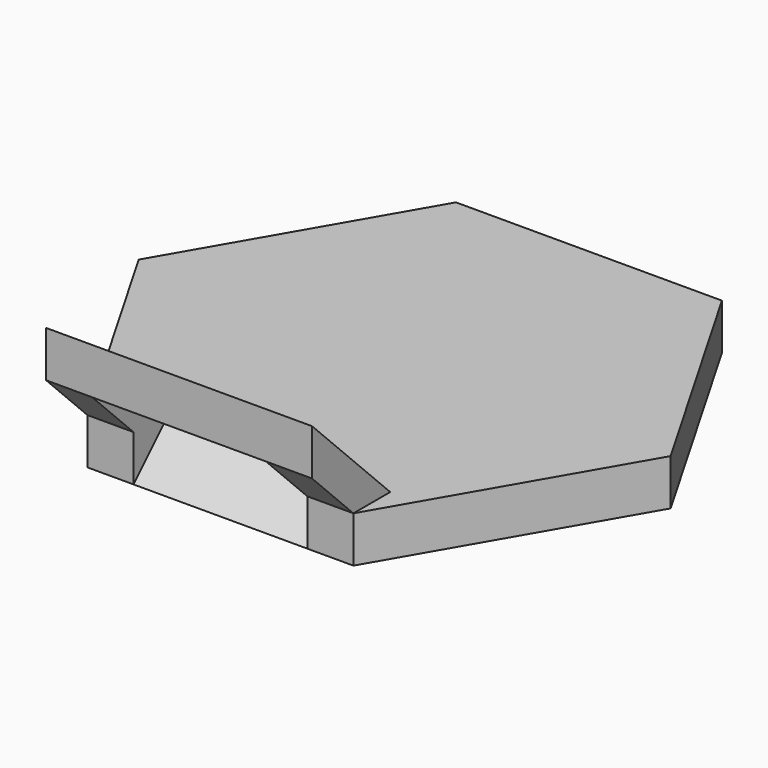
from build123d import *

# Parameters (mm, degrees)
F1_DEPTH = 2
F4_DEPTH = 11.54701
F5_W     = 7.54701
F5_H     = 6
F6_DEPTH = 25
F8_DEPTH = 7.54701


# Not quite as in the source:
# - the program builds the solid bodies; features that only make, move or delete a surface that nothing else refers to are left out


with BuildPart() as f1:
    # F0 (on Top) → F1 (new body)
    with BuildSketch(Plane.XY):
        Polygon((-3.7735026919, -10), (5.7735026919, -10), (11.5470053838, 0), (5.7735026919, 10), (0, 10), (-5.7735026919, 10), (-11.5470053838, 0), (-6.7735026919, -8.2679491924), (-5.7735026919, -10), align=None)
    extrude(amount=-F1_DEPTH)

    # F3 (on face) → F4 (join)
    with BuildSketch(Plane.YZ.offset(-5.7735026919)):
        Polygon((-10, 2), (-10, 0), (-8, 0), align=None)
        Polygon((-12.2426406871, 2.2426406871), (-10, 0), (-10, 2), (-12.2426406871, 4.2426406871), align=None)
    extrude(amount=F4_DEPTH)

    # F5 (on face) → F6 (cut)
    with BuildSketch(Plane(origin=(0, -4, -4), x_dir=(-1, 0, 0), z_dir=(0, 0.7071067812, 0.7071067812))):
        with Locations((-2.3081e-06, 8.6568542495)):
            Rectangle(F5_W, F5_H)
    extrude(amount=-F6_DEPTH, mode=Mode.SUBTRACT)

    # F7 (on face) → F8 (join, through all)
    with BuildSketch(Plane.YZ.offset(-3.7735026919)):
        Polygon((-12.2426406871, 4.2426406871), (-12.2426406871, 2.2426406871), (-10.2426406871, 2.2426406871), align=None)
    extrude(amount=F8_DEPTH)


solid = f1.part
